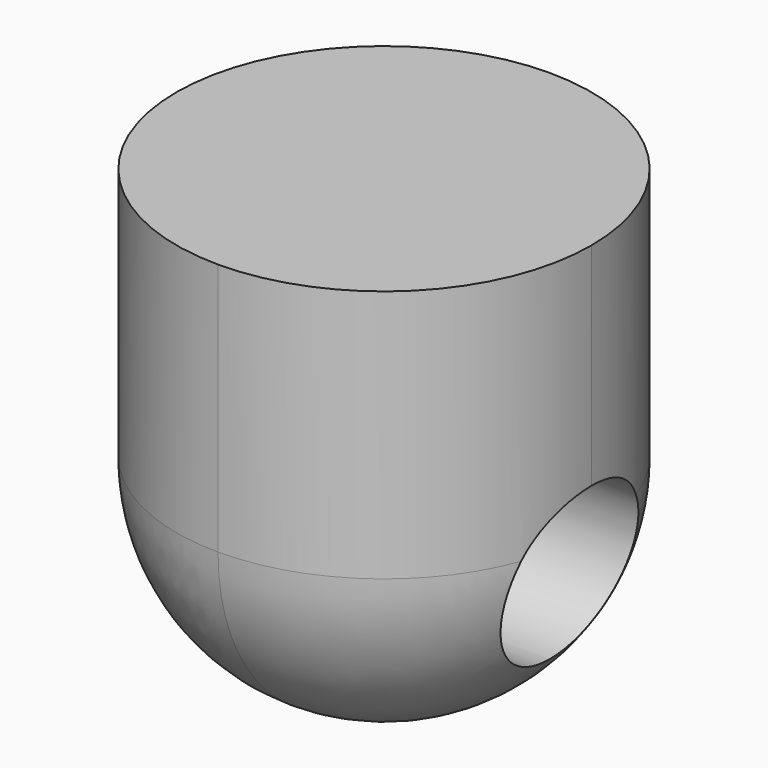
from build123d import *

# Parameters (mm, degrees)
F0_W         = 50
F0_H         = 50
F1_DEPTH     = 55.5
F2_R         = 10
F3_DEPTH     = 25
F4_R         = 24.99999
F5_T1_DEPTH  = 155.50001
F5_T3_DEPTH  = 125.00002
F5_T6_ANGLE  = 90
F5_T8_ANGLE  = 90
F5_T10_ANGLE = 90
F5_T12_ANGLE = 90


# Not quite as in the source:
# - a fillet or chamfer that OpenCascade refuses, or shapes differently, is made with other operations: its cross-section is extruded or revolved along the edge and cut away or added
# - a fillet or chamfer is up to 0.001 mm smaller than in the source, because OpenCascade refuses the exact size


with BuildPart() as f1:
    # F0 (on Top) → F1 (new body)
    with BuildSketch(Plane.XY):
        Rectangle(F0_W, F0_H)
    extrude(amount=F1_DEPTH)

    # F2 (on face) → F3 (cut)
    with BuildSketch(Plane.YZ.offset(25)):
        with Locations((0, 20)):
            Circle(F2_R)
    extrude(amount=-F3_DEPTH, mode=Mode.SUBTRACT)

    # F4 (radius 25 in the source; OpenCascade refuses exactly that, so slightly less here)
    f4_edges = [f1.edges().sort_by_distance(p)[0] for p in [
        (0, -25, 0),
        (0, 25, 0),
    ]]
    fillet(f4_edges, radius=F4_R)

    # F5: fillet of radius 25 on 2 edges, made by hand

    # F5_s2 → F5_t1 (cut)
    with BuildSketch(Plane.XY.offset(-37.50001)):
        with BuildLine():
            ThreePointArc((25, 0), (17.6776695297, -17.6776695297), (0, -25))
            Line((0, -25), (25, -25))
            Line((25, -25), (25, 0))
        make_face()
        with BuildLine():
            ThreePointArc((-25, 0), (-17.6776695297, -17.6776695297), (0, -25))
            Line((0, -25), (-25, -25))
            Line((-25, -25), (-25, 0))
        make_face()
        with BuildLine():
            ThreePointArc((0, 25), (-17.6776695297, 17.6776695297), (-25, 0))
            Line((-25, 0), (-25, 25))
            Line((-25, 25), (0, 25))
        make_face()
        with BuildLine():
            ThreePointArc((0, 25), (17.6776695297, 17.6776695297), (25, 0))
            Line((25, 0), (25, 25))
            Line((25, 25), (0, 25))
        make_face()
    extrude(amount=F5_T1_DEPTH, mode=Mode.SUBTRACT)

    # F5_s4 → F5_t3 (cut)
    with BuildSketch(Plane.XZ.offset(-62.50001)):
        with BuildLine():
            ThreePointArc((-25, 25), (-17.6776695297, 7.3223304703), (0, 0))
            Line((0, 0), (-25, 0))
            Line((-25, 0), (-25, 25))
        make_face()
        with BuildLine():
            ThreePointArc((25, 25), (17.6776695297, 7.3223304703), (0, 0))
            Line((0, 0), (25, 0))
            Line((25, 0), (25, 25))
        make_face()
    extrude(amount=F5_T3_DEPTH, mode=Mode.SUBTRACT)

    # F5_s5 → F5_t6 (revolve, cut)
    with BuildSketch(Plane.XZ.offset(1e-05)):
        with BuildLine():
            ThreePointArc((-25, 24.99999), (-17.6776659941, 7.3223269348), (0, 0))
            Line((0, 0), (-25, 0))
            Line((-25, 0), (-25, 24.99999))
        make_face()
    revolve(axis=Axis((-25, -1e-05, 24.99999), (-1, 0, 0)), revolution_arc=F5_T6_ANGLE, mode=Mode.SUBTRACT)

    # F5_s7 → F5_t8 (revolve, cut)
    with BuildSketch(Plane.XY.offset(24.99999)):
        with BuildLine():
            ThreePointArc((0, 25), (-17.6776659941, 17.6776730652), (-25, 1e-05))
            Line((-25, 1e-05), (-25, 25))
            Line((-25, 25), (0, 25))
        make_face()
    revolve(axis=Axis((-25, 1e-05, 24.99999), (-1, 0, 0)), revolution_arc=F5_T8_ANGLE, mode=Mode.SUBTRACT)

    # F5_s9 → F5_t10 (revolve, cut)
    with BuildSketch(Plane.XZ.offset(1e-05)):
        with BuildLine():
            ThreePointArc((25, 24.99999), (17.6776659941, 7.3223269348), (0, 0))
            Line((0, 0), (25, 0))
            Line((25, 0), (25, 24.99999))
        make_face()
    revolve(axis=Axis((25, -1e-05, 24.99999), (-1, 0, 0)), revolution_arc=F5_T10_ANGLE, mode=Mode.SUBTRACT)

    # F5_s11 → F5_t12 (revolve, cut)
    with BuildSketch(Plane.XY.offset(24.99999)):
        with BuildLine():
            ThreePointArc((25, 1e-05), (17.6776659941, 17.6776730652), (0, 25))
            Line((0, 25), (25, 25))
            Line((25, 25), (25, 1e-05))
        make_face()
    revolve(axis=Axis((25, 1e-05, 24.99999), (-1, 0, 0)), revolution_arc=F5_T12_ANGLE, mode=Mode.SUBTRACT)


solid = f1.part
